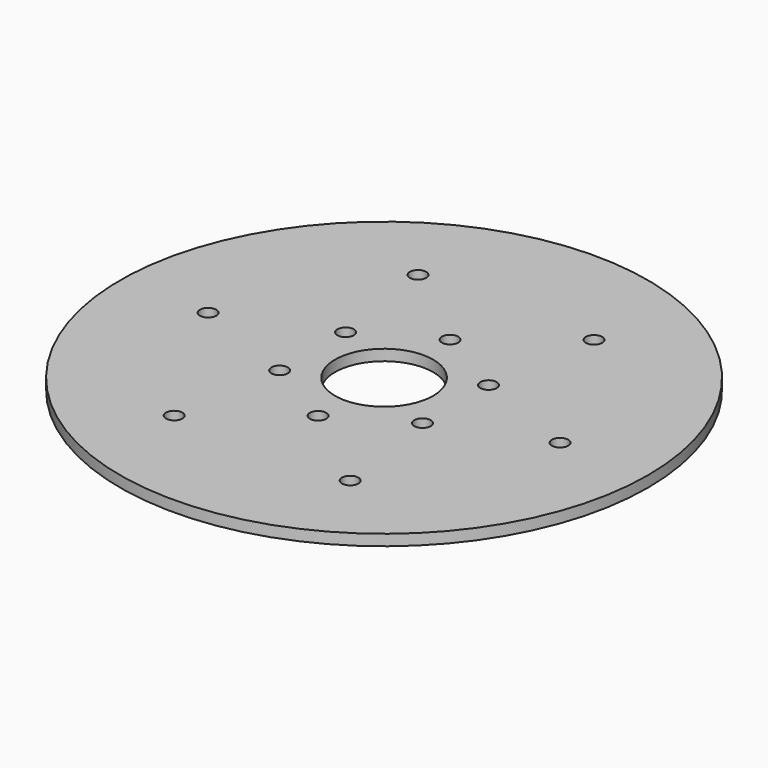
from build123d import *

# Parameters (mm, degrees)
F0_R            = 76.2
F0_R_2          = 14.1605
F1_DEPTH        = 3.175
F2_R            = 2.3622
F3_DEPTH        = 3.176
F3_COPIES_COUNT = 6


# Not quite as in the source:
# - a pattern or mirror of a feature is missing from the dataset's text; its kind, count and spacing are read off the source's solid


with BuildPart() as f1:
    # F0 (on Top) → F1 (new body)
    with BuildSketch(Plane.XY):
        Circle(F0_R)
        Circle(F0_R_2, mode=Mode.SUBTRACT)
    extrude(amount=F1_DEPTH)

    # F2 (on face) → F3 (cut, through all)
    with BuildSketch(Plane.XY.offset(3.175)):
        with Locations((0, 23.8125)):
            Circle(F2_R)
        with Locations((25.4, 43.9940905122)):
            Circle(F2_R)
    f3 = extrude(amount=-F3_DEPTH, mode=Mode.SUBTRACT)

    # F3_copies: F3 ×6 about axis
    f3_copies_axis = Axis((0, 0, 0), (0, 0, 1))
    for i in range(1, F3_COPIES_COUNT):
        add(f3.rotate(f3_copies_axis, i * 360 / F3_COPIES_COUNT), mode=Mode.SUBTRACT)


solid = f1.part
